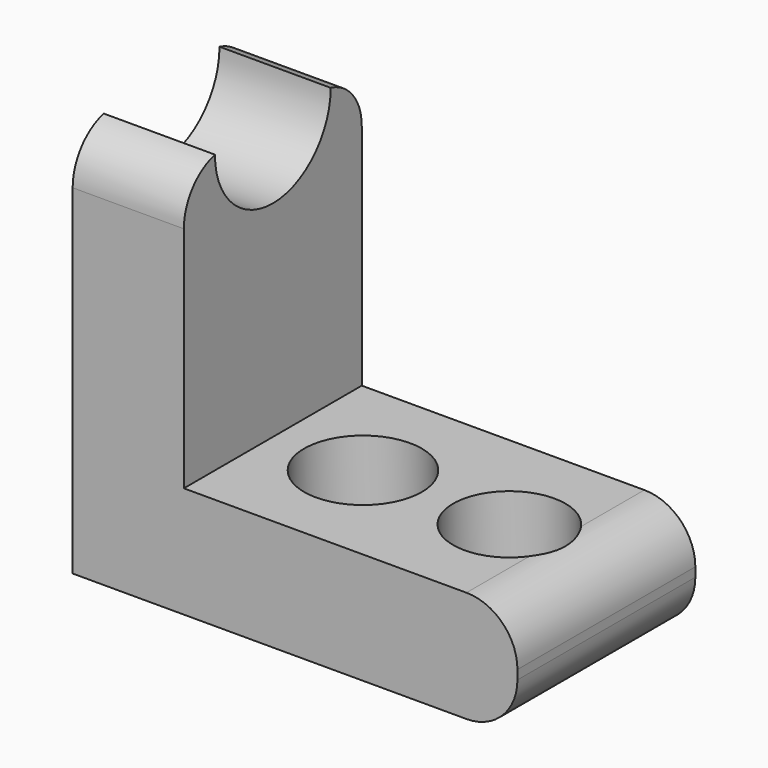
from build123d import *

# Parameters (mm, degrees)
F1_DEPTH    = 50.8
F3_DEPTH    = 25.4
F4_R        = 13.4399022195
F4_R_2      = 12.8262913295
F5_DEPTH    = 50.8
F6_T1_DEPTH = 81.9737109729
F6_T3_DEPTH = 109.0549732601


# Not quite as in the source:
# - a fillet or chamfer that OpenCascade refuses, or shapes differently, is made with other operations: its cross-section is extruded or revolved along the edge and cut away or added


with BuildPart() as f1:
    # F0 (on Front) → F1 (new body)
    with BuildSketch(Plane.XZ):
        Polygon((-46.0024929225, 49.746170783), (-46.0024929225, -39.153829217), (55.5975070775, -39.153829217), (55.5975070775, -13.753829217), (-20.6024929225, -13.753829217), (-20.6024929225, 49.746170783), align=None)
    extrude(amount=F1_DEPTH)

    # F2 (on face) → F3 (cut)
    with BuildSketch(Plane.YZ.offset(-20.6024929225)):
        with BuildLine():
            Line((-38.1, 49.746170783), (-41.9279053914, 49.746170783))
            ThreePointArc((-41.9279053914, 49.746170783), (-25.4, 33.2182653916), (-8.8720946086, 49.746170783))
            Line((-8.8720946086, 49.746170783), (-12.7, 49.746170783))
            Line((-12.7, 49.746170783), (-38.1, 49.746170783))
        make_face()
    extrude(amount=-F3_DEPTH, mode=Mode.SUBTRACT)

    # F4 (on face) → F5 (cut)
    with BuildSketch(Plane.XY.offset(-13.753829217)):
        with Locations((0, -25.4)):
            Circle(F4_R)
        with Locations((33.4277749062, -25.4)):
            Circle(F4_R_2)
    extrude(amount=-F5_DEPTH, mode=Mode.SUBTRACT)

    # F6: fillet of radius 11.650994652 on 4 edges, made by hand

    # F6_s2 → F6_t1 (cut)
    with BuildSketch(Plane.YZ.offset(-74.289348409)):
        with BuildLine():
            ThreePointArc((-41.9279053914, 49.746170783), (-48.3175010241, 45.6206123682), (-50.8, 38.4314285885))
            Line((-50.8, 38.4314285885), (-50.8, 49.746170783))
            Line((-50.8, 49.746170783), (-41.9279053914, 49.746170783))
        make_face()
        with BuildLine():
            ThreePointArc((0, 38.4314285885), (-2.4824989759, 45.6206123682), (-8.8720946086, 49.746170783))
            Line((-8.8720946086, 49.746170783), (0, 49.746170783))
            Line((0, 49.746170783), (0, 38.4314285885))
        make_face()
    extrude(amount=F6_T1_DEPTH, mode=Mode.SUBTRACT)

    # F6_s4 → F6_t3 (cut)
    with BuildSketch(Plane.XZ.offset(-29.12748663)):
        with BuildLine():
            ThreePointArc((43.9465124254, -13.753829217), (52.1850097514, -17.166326543), (55.5975070775, -25.404823869))
            Line((55.5975070775, -25.404823869), (55.5975070775, -13.753829217))
            Line((55.5975070775, -13.753829217), (43.9465124254, -13.753829217))
        make_face()
        with BuildLine():
            ThreePointArc((43.9465124254, -39.153829217), (52.1850097514, -35.741331891), (55.5975070775, -27.5028345649))
            Line((55.5975070775, -27.5028345649), (55.5975070775, -39.153829217))
            Line((55.5975070775, -39.153829217), (43.9465124254, -39.153829217))
        make_face()
    extrude(amount=F6_T3_DEPTH, mode=Mode.SUBTRACT)


solid = f1.part
